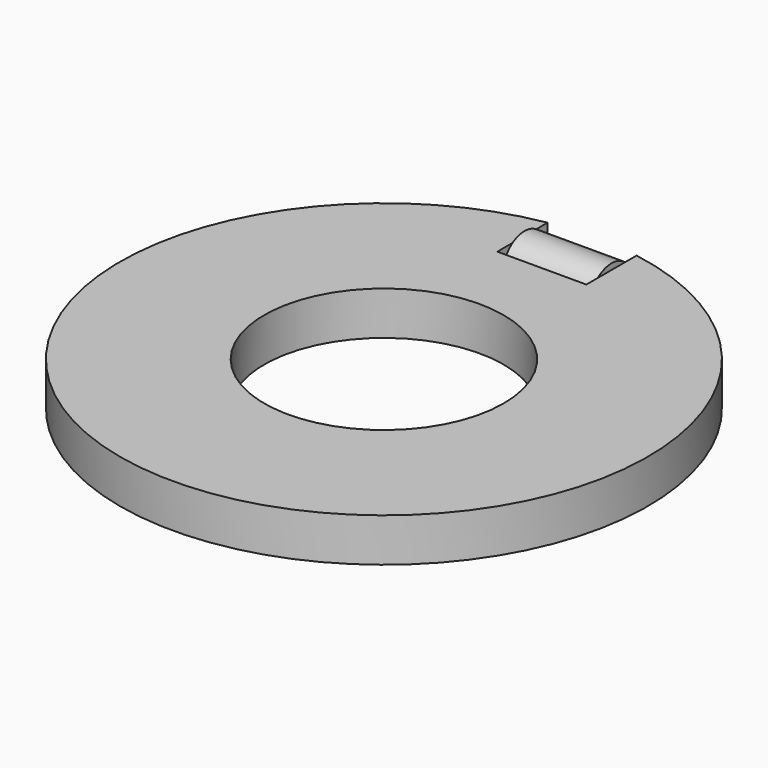
from build123d import *

# Parameters (mm, degrees)
F0_R     = 48.5166715587
F0_R_2   = 22
F1_DEPTH = 8
F3_DEPTH = 25.4
F8_R     = 5.0035531794
F9_DEPTH = 8


# Not quite as in the source:
# - a pattern or mirror of a feature is missing from the dataset's text; its kind, count and spacing are read off the source's solid


with BuildPart() as f1:
    # F0 (on Top) → F1 (new body)
    with BuildSketch(Plane.XY):
        Circle(F0_R)
        Circle(F0_R_2, mode=Mode.SUBTRACT)
    extrude(amount=F1_DEPTH)

    # F2 (on Top) → F3 (cut)
    with BuildSketch(Plane.XY):
        Polygon((-8.1793928312, 54.083118853), (-8.1793928312, 47.8222223663), (-8.1793928312, 36.2803220355), (0, 36.2803220355), (8.1793928312, 36.2803220355), (8.1793928312, 54.083118853), align=None)
    extrude(amount=F3_DEPTH, mode=Mode.SUBTRACT)

    # F6 (on offset) → F7 (revolve)
    with BuildSketch(Plane(origin=(0, 42.2803220355, 0), x_dir=(-1, 0, 0), z_dir=(0, 1, 0))):
        with BuildLine():
            ThreePointArc((6.6793928312, 4), (7.1187326594, 2.9393398282), (8.1793928312, 2.5))
            Line((8.1793928312, 2.5), (8.1793928312, 4))
            Line((8.1793928312, 4), (6.6793928312, 4))
        make_face()
    f7 = revolve(axis=Axis((-2.9829649384, 42.2803220355, 4), (1, 0, 0)))

    # F7_copies: F7 across plane
    add(f7.mirror(Plane(origin=(0, 0, 0), x_dir=(0, 0, 1), z_dir=(1, 0, 0))))


with BuildPart() as f9:
    # F8 (on Right) → F9 (new body, symmetric)
    with BuildSketch(Plane.YZ):
        with Locations((42.2803220355, 3.9445757866)):
            Circle(F8_R)
    extrude(amount=F9_DEPTH, both=True)

    # F6 (on offset) → F10 (revolve, cut)
    with BuildSketch(Plane(origin=(0, 42.2803220355, 0), x_dir=(-1, 0, 0), z_dir=(0, 1, 0))):
        with BuildLine():
            ThreePointArc((8.1793928312, 5.8), (6.906600625, 5.2727922061), (6.3793928312, 4))
            Line((6.3793928312, 4), (6.6793928312, 4))
            ThreePointArc((6.6793928312, 4), (7.1187326594, 5.0606601718), (8.1793928312, 5.5))
            Line((8.1793928312, 5.5), (8.1793928312, 5.8))
        make_face()
        with BuildLine():
            Line((6.6793928312, 4), (8.1793928312, 4))
            Line((8.1793928312, 4), (8.1793928312, 5.5))
            ThreePointArc((8.1793928312, 5.5), (7.1187326594, 5.0606601718), (6.6793928312, 4))
        make_face()
    f10 = revolve(axis=Axis((-2.9829649384, 42.2803220355, 4), (1, 0, 0)), mode=Mode.SUBTRACT)

    # F10_copies: F10 across plane
    add(f10.mirror(Plane(origin=(0, 0, 0), x_dir=(0, 0, 1), z_dir=(1, 0, 0))), mode=Mode.SUBTRACT)


solid = Compound([f1.part, f9.part])
